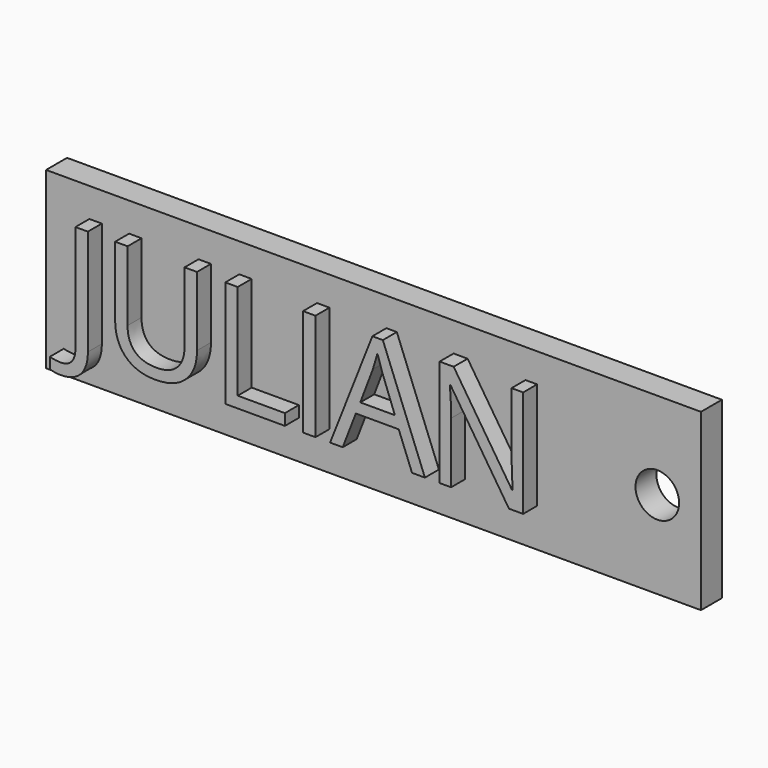
from build123d import *

# Parameters (mm, degrees)
F0_W         = 75
F0_H         = 20
F0_R         = 2.5
F1_DEPTH     = 3
F2_TEXT_SIZE = 17.1568629513
F3_DEPTH     = 2


# Not quite as in the source:
# - Text() gives the source's letters only with a copy of the font that has no kerning and outlines rounded to 1/6400 em; it was checked with that copy


with BuildPart() as f1:
    # F0 (on Front) → F1 (new body)
    with BuildSketch(Plane.XZ):
        with Locations((37.5, -10)):
            Rectangle(F0_W, F0_H)
        with Locations((70, -10)):
            Circle(F0_R, mode=Mode.SUBTRACT)
    extrude(amount=F1_DEPTH)

    # F2 (on face) → F3 (join)
    with BuildSketch(Plane.XZ.offset(3)):
        with Locations((3.3689851407, -15.5815510079)):
            Text('JULIAN', F2_TEXT_SIZE, font='Open Sans', text_align=(TextAlign.LEFT, TextAlign.BOTTOM))
    extrude(amount=F3_DEPTH)


solid = f1.part
